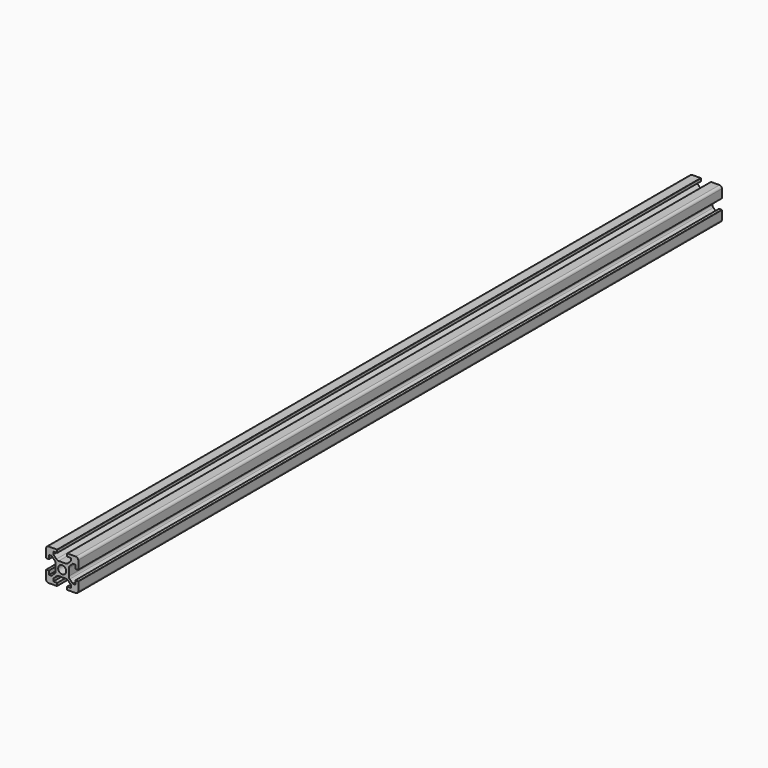
from build123d import *

# Parameters (mm, degrees)
F0_R     = 2.5
F1_DEPTH = 500
F2_R     = 1.5
F3_R     = 2
F4_R     = 0.2


# Not quite as in the source:
# - a feature names something its author has since deleted; it is built from what else it names


with BuildPart() as f1:
    # F0 (on Front) → F1 (new body)
    with BuildSketch(Plane.XZ):
        Polygon((-3.1, 10), (-10, 10), (-10, 3.1), (-8.2, 3.1), (-8.2, 5.5), (-6.6, 5.5), (-4.1, 3), (-4.1, -3), (-6.6, -5.5), (-8.2, -5.5), (-8.2, -3.1), (-10, -3.1), (-10, -10), (-3.1, -10), (-3.1, -8.2), (-5.5, -8.2), (-5.5, -6.6), (-3, -4.1), (0, -4.1), (3, -4.1), (5.5, -6.6), (5.5, -8.2), (3.1, -8.2), (3.1, -10), (10, -10), (10, -3.1), (8.2, -3.1), (8.2, -5.5), (6.6, -5.5), (4.1, -3), (4.1, 3), (6.6, 5.5), (8.2, 5.5), (8.2, 3.1), (10, 3.1), (10, 10), (3.1, 10), (3.1, 8.2), (5.5, 8.2), (5.5, 6.6), (3, 4.1), (0, 4.1), (-3, 4.1), (-5.5, 6.6), (-5.5, 8.2), (-3.1, 8.2), align=None)
        Circle(F0_R, mode=Mode.SUBTRACT)
    extrude(amount=F1_DEPTH)

    # F2
    f2_edges = [f1.edges().sort_by_distance(p)[0] for p in [
        (-10, -250, 10),
        (10, -250, 10),
        (10, -250, -10),
        (-10, -250, -10),
    ]]
    fillet(f2_edges, radius=F2_R)

    # F3
    f3_edges = [f1.edges().sort_by_distance(p)[0] for p in [
        (-4.1, -250, 3),
        (-4.1, -250, -3),
        (3, -250, 4.1),
        (-3, -250, 4.1),
        (4.1, -250, 3),
        (4.1, -250, -3),
        (3, -250, -4.1),
        (-3, -250, -4.1),
    ]]
    fillet(f3_edges, radius=F3_R)

    # F4
    f4_edges = [f1.edges().sort_by_distance(p)[0] for p in [
        (-10, -250, 3.1),
        (-3.1, -250, -10),
        (3.1, -250, -10),
        (10, -250, -3.1),
        (10, -250, 3.1),
        (-10, -250, -3.1),
        (3.1, -250, 10),
        (-3.1, -250, 10),
    ]]
    fillet(f4_edges, radius=F4_R)


solid = f1.part
